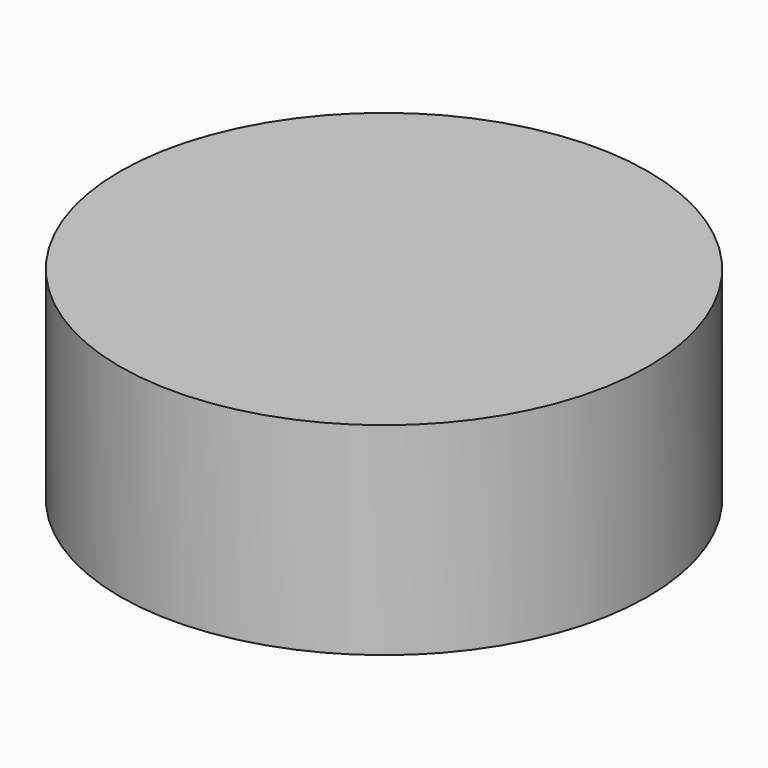
from build123d import *

# Parameters (mm, degrees)
F0_R     = 41.75
F1_DEPTH = 32


# Not quite as in the source:
# - a feature of the source that left no trace in its solid (it failed there, or was rolled back) is left out
# - the program builds the solid bodies; features that only make, move or delete a surface that nothing else refers to are left out


with BuildPart() as f1:
    # F0 (on Top) → F1 (new body)
    with BuildSketch(Plane.XY):
        Circle(F0_R)
    extrude(amount=F1_DEPTH)


with BuildPart() as f1_1:
    # F3: moved
    add(f1.part.moved(Location((0, 0, 30))))


solid = f1_1.part
